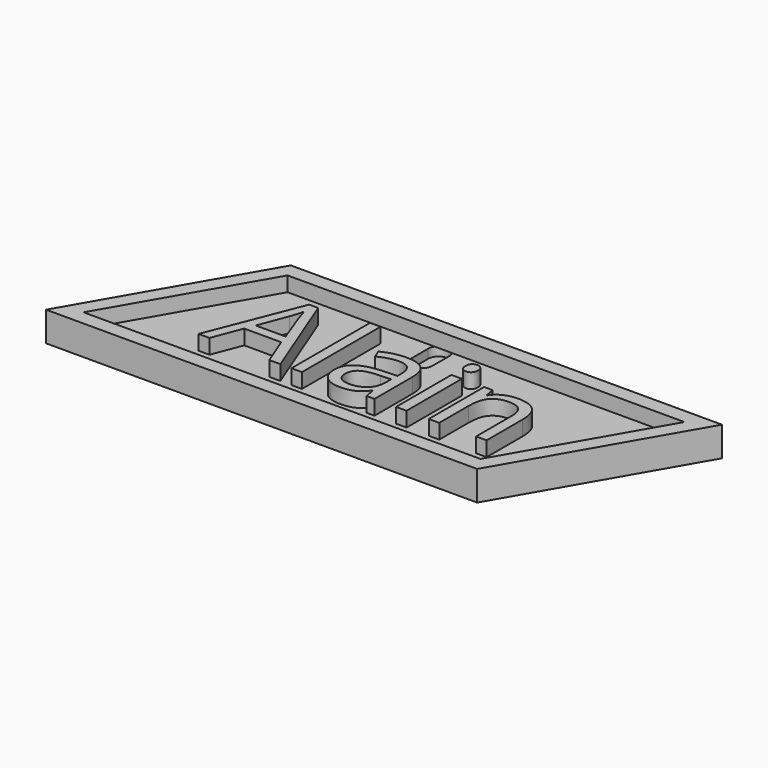
from build123d import *

# Parameters (mm, degrees)
F1_DEPTH     = 10
F3_DEPTH     = 5
F4_TEXT_SIZE = 43.6115843271
F5_DEPTH     = 5
F8_DEPTH     = 3


# Not quite as in the source:
# - Text() gives the source's letters only with a copy of the font that has no kerning and outlines rounded to 1/6400 em; it was checked with that copy


with BuildPart() as f1:
    # F0 (on Top) → F1 (new body)
    with BuildSketch(Plane.XY):
        Polygon((90, 30), (-55.4385079217, 30), (-90, -30), (55.4385079217, -30), align=None)
    extrude(amount=F1_DEPTH)

    # F2 (on face) → F3 (cut)
    with BuildSketch(Plane.XY.offset(10)):
        Polygon((81.3496836172, 25), (-52.5484402186, 25), (-81.3496836172, -25), (52.5484402186, -25), align=None)
    extrude(amount=-F3_DEPTH, mode=Mode.SUBTRACT)

    # F4 (on face) → F5 (join)
    with BuildSketch(Plane.XY.offset(5)):
        with Locations((-50, -15.7001703578)):
            Text('Alain', F4_TEXT_SIZE, font='Open Sans', text_align=(TextAlign.LEFT, TextAlign.BOTTOM))
    extrude(amount=F5_DEPTH)

    # F7 (on offset) → F8 (cut)
    with BuildSketch(Plane.XY.offset(5)):
        with BuildLine():
            Line((3.5, 16), (3.5, 23))
            ThreePointArc((3.5, 23), (0, 26.5), (-3.5, 23))
            Line((-3.5, 23), (-3.5, 16))
            ThreePointArc((-3.5, 16), (0, 12.5), (3.5, 16))
        make_face()
    extrude(amount=-F8_DEPTH, mode=Mode.SUBTRACT)


solid = f1.part
